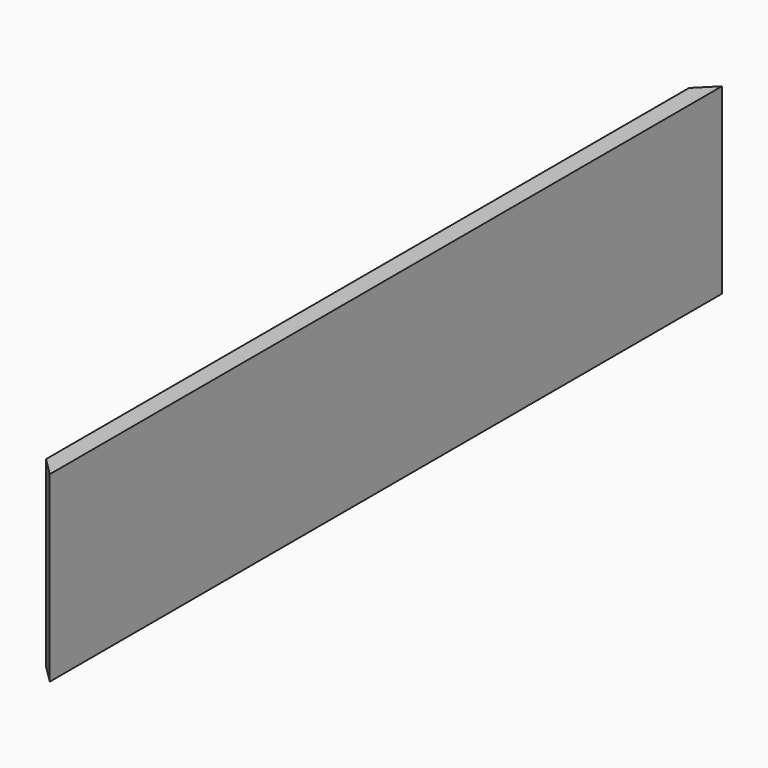
from build123d import *

# Parameters (mm, degrees)
F0_W        = 19.05
F0_H        = 190.5
F1_DEPTH    = 457.2
F2_T1_DEPTH = 386.462243683


# Not quite as in the source:
# - a fillet or chamfer that OpenCascade refuses, or shapes differently, is made with other operations: its cross-section is extruded or revolved along the edge and cut away or added


with BuildPart() as f1:
    # F0 (on Front) → F1 (new body, symmetric)
    with BuildSketch(Plane.XZ):
        Rectangle(F0_W, F0_H)
    extrude(amount=F1_DEPTH, both=True)

    # F2: chamfer of 38.1 on 2 edges, made by hand

    # F2_s2 → F2_t1 (cut)
    with BuildSketch(Plane.XY.offset(-193.2311218415)):
        Polygon((-9.525, 419.1), (28.575, 457.2), (-9.525, 457.2), align=None)
        Polygon((-9.525, -419.1), (28.575, -457.2), (-9.525, -457.2), align=None)
    extrude(amount=F2_T1_DEPTH, mode=Mode.SUBTRACT)


solid = f1.part
